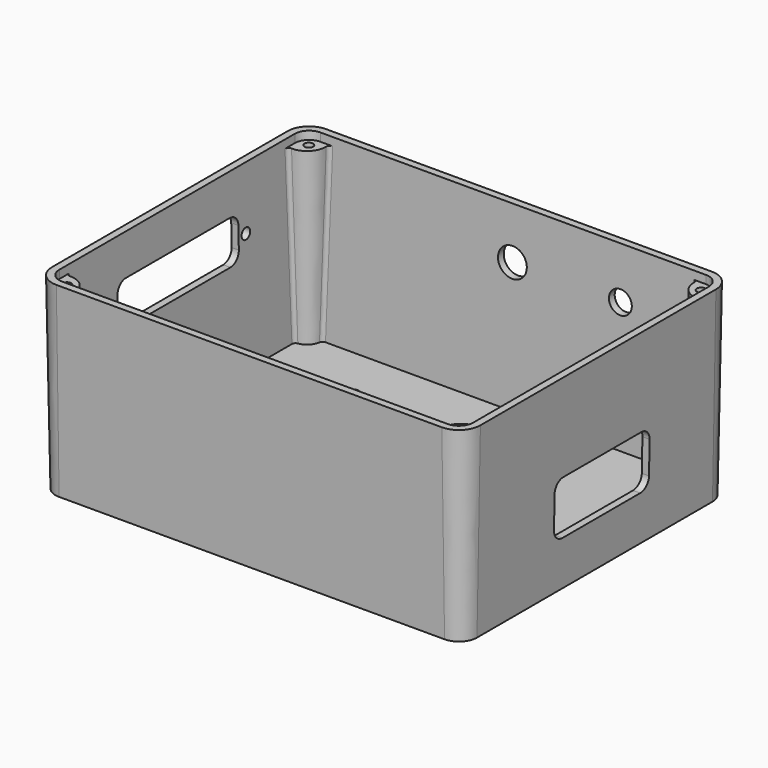
from build123d import *

# Parameters (mm, degrees)
F1_DEPTH                  = 52.25
F1_TAPER                  = -1.05
F2_T                      = 2
F4_D                      = 3
F4_CSINK_D                = 6.5
F4_CSINK_ANGLE            = 90
F6_REACH                  = 95.7577764887
F7_R                      = 1.5
F8_REACH                  = 103.1892979036
F9_R                      = 4
F9_R_2                    = 3.175
F10_REACH                 = 58.1723470669
F12_DEPTH                 = 48
DRAFT_F12_DRAFTED_ANGLE   = -1.5
DRAFT_F12_2_DRAFTED_ANGLE = -1.5
DRAFT_F12_3_DRAFTED_ANGLE = -1.5
DRAFT_F12_4_DRAFTED_ANGLE = -1.5
F13_R                     = 1
F15_D                     = 2.4
F15_DEPTH                 = 8
F15_TIP                   = 0.7210327428


# Not quite as in the source:
# - an extrude with a draft is written as a straight extrude whose walls are then drafted
# - a shell that OpenCascade refuses in one call is made with other operations: the cavity is built on its own and cut out


with BuildPart() as f1:
    # F0 (on Top) → F1 (new body)
    with BuildSketch(Plane.XY):
        with BuildLine():
            ThreePointArc((58.55, 40.9), (57.0855339059, 44.4355339059), (53.55, 45.9))
            Line((53.55, 45.9), (-53.55, 45.9))
            ThreePointArc((-53.55, 45.9), (-57.0855339059, 44.4355339059), (-58.55, 40.9))
            Line((-58.55, 40.9), (-58.55, -40.9))
            ThreePointArc((-58.55, -40.9), (-57.0855339059, -44.4355339059), (-53.55, -45.9))
            Line((-53.55, -45.9), (53.55, -45.9))
            ThreePointArc((53.55, -45.9), (57.0855339059, -44.4355339059), (58.55, -40.9))
            Line((58.55, -40.9), (58.55, 40.9))
        make_face()
    extrude(amount=F1_DEPTH, taper=F1_TAPER)

    # F2: shell of thickness 2, made by hand


with BuildPart() as f2_core1:
    # F2_t2: copy of F1
    add(f1.part)

    # the walls: a layer under each face that stays
    f2_faces = [f2_core1.faces().sort_by_distance(p)[0] for p in [
        (59.028819234, 0, 26.125),
        (57.4241102332, 44.7741102332, 26.125),
        (0, 46.378819234, 26.125),
        (-57.4241102332, 44.7741102332, 26.125),
        (-59.028819234, 0, 26.125),
        (-57.4241102332, -44.7741102332, 26.125),
        (0, -46.378819234, 26.125),
        (57.4241102332, -44.7741102332, 26.125),
        (0, 0, 0),
    ]]
    thicken(f2_faces, amount=-F2_T, mode=Mode.SUBTRACT)


with BuildPart() as f1_1:
    add(f1.part)

    # what is left inside the walls is the cavity
    f2_cavity = [f2_core1.part.solids().sort_by_distance(p)[0] for p in [
        (0, -14.952434, 52.23),
    ]]
    add(f2_cavity, mode=Mode.SUBTRACT)

    # F4 (through all)
    with Locations(Plane(origin=(0, 0, 0), x_dir=(1, 0, 0), z_dir=(0, 0, -1))):
        with Locations((50.05, 21.25), (50.05, -29.25), (-31.865, -29.25), (-31.865, 21.25)):
            CounterSinkHole(F4_D / 2, F4_CSINK_D / 2, counter_sink_angle=F4_CSINK_ANGLE)

    f6_end = f1_1.faces().sort_by_distance((59.028819234, 0, 26.125))[0]
    # F5 (on Right) → F6 (cut, up to a face of the model that its end follows)
    with BuildSketch(Plane.YZ):
        with BuildLine():
            Line((-11.5, 12.5), (15.5, 12.5))
            ThreePointArc((15.5, 12.5), (17.6213203436, 13.3786796564), (18.5, 15.5))
            Line((18.5, 15.5), (18.5, 24.5))
            ThreePointArc((18.5, 24.5), (17.6213203436, 26.6213203436), (15.5, 27.5))
            Line((15.5, 27.5), (-11.5, 27.5))
            ThreePointArc((-11.5, 27.5), (-13.6213203436, 26.6213203436), (-14.5, 24.5))
            Line((-14.5, 24.5), (-14.5, 15.5))
            ThreePointArc((-14.5, 15.5), (-13.6213203436, 13.3786796564), (-11.5, 12.5))
        make_face()
    f6_long = extrude(amount=F6_REACH, mode=Mode.PRIVATE)
    add(split(f6_long, bisect_by=f6_end, keep=Keep.BOTTOM, mode=Mode.PRIVATE), mode=Mode.SUBTRACT)

    f8_end = f1_1.faces().sort_by_distance((-59.028819234, 0, 26.125))[0]
    # F7 (on Right) → F8 (cut, up to a face of the model that its end follows)
    with BuildSketch(Plane.YZ):
        with BuildLine():
            ThreePointArc((21, 38), (20.1213203436, 40.1213203436), (18, 41))
            Line((18, 41), (-18, 41))
            ThreePointArc((-18, 41), (-20.1213203436, 40.1213203436), (-21, 38))
            Line((-21, 38), (-21, 32))
            ThreePointArc((-21, 32), (-20.1213203436, 29.8786796564), (-18, 29))
            Line((-18, 29), (18, 29))
            ThreePointArc((18, 29), (20.1213203436, 29.8786796564), (21, 32))
            Line((21, 32), (21, 38))
        make_face()
        with Locations((-23.52, 35)):
            Circle(F7_R)
        with Locations((23.52, 35)):
            Circle(F7_R)
    f8_long = extrude(amount=-F8_REACH, mode=Mode.PRIVATE)
    add(split(f8_long, bisect_by=f8_end, keep=Keep.BOTTOM, mode=Mode.PRIVATE), mode=Mode.SUBTRACT)

    f10_end = f1_1.faces().sort_by_distance((0, 46.378819234, 26.125))[0]
    # F9 (on Front) → F10 (cut, up to a face of the model that its end follows)
    with BuildSketch(Plane.XZ):
        with Locations((0, 38)):
            Circle(F9_R)
        with Locations((30, 38)):
            Circle(F9_R_2)
    f10_long = extrude(amount=-F10_REACH, mode=Mode.PRIVATE)
    add(split(f10_long, bisect_by=f10_end, keep=Keep.BOTTOM, mode=Mode.PRIVATE), mode=Mode.SUBTRACT)


with BuildPart() as f12_drafted:
    # F11 (on face) → F12 (new body)
    with BuildSketch(Plane.XY.offset(2)):
        with BuildLine():
            Line((-56.5863201302, 40.9), (-56.5863201302, 39.7053273134))
            ThreePointArc((-56.5863201302, 39.7053273134), (-53.5198083649, 40.8698083649), (-52.3553273134, 43.9363201302))
            Line((-52.3553273134, 43.9363201302), (-53.55, 43.9363201302))
            ThreePointArc((-53.55, 43.9363201302), (-55.6970025539, 43.0470025539), (-56.5863201302, 40.9))
        make_face()
    extrude(amount=F12_DEPTH)

    # draft_F12_drafted
    draft_f12_drafted_walls = [f12_drafted.faces().sort_by_distance(p)[0] for p in [
        (-56.5863201302, 40.3026636567, 34),
        (-53.5198083649, 40.8698083649, 34),
        (-52.9526636567, 43.9363201302, 34),
        (-55.6970025539, 43.0470025539, 34),
    ]]
    draft(draft_f12_drafted_walls, neutral_plane=Plane.XY.offset(2), angle=DRAFT_F12_DRAFTED_ANGLE)


with BuildPart() as f1_2:
    add(f1_1.part)

    # join_F12_drafted: union F12_drafted
    add(f12_drafted.part)


with BuildPart() as f12_2_drafted:
    # F11 (on face) → F12, piece 2 (new body)
    with BuildSketch(Plane.XY.offset(2)):
        with BuildLine():
            Line((53.55, 43.9363201302), (52.3553273134, 43.9363201302))
            ThreePointArc((52.3553273134, 43.9363201302), (53.5198083649, 40.8698083649), (56.5863201302, 39.7053273134))
            Line((56.5863201302, 39.7053273134), (56.5863201302, 40.9))
            ThreePointArc((56.5863201302, 40.9), (55.6970025539, 43.0470025539), (53.55, 43.9363201302))
        make_face()
    extrude(amount=F12_DEPTH)

    # draft_F12_2_drafted
    draft_f12_2_drafted_walls = [f12_2_drafted.faces().sort_by_distance(p)[0] for p in [
        (52.9526636567, 43.9363201302, 34),
        (53.5198083649, 40.8698083649, 34),
        (56.5863201302, 40.3026636567, 34),
        (55.6970025539, 43.0470025539, 34),
    ]]
    draft(draft_f12_2_drafted_walls, neutral_plane=Plane.XY.offset(2), angle=DRAFT_F12_2_DRAFTED_ANGLE)


with BuildPart() as f1_3:
    add(f1_2.part)

    # join_F12_2_drafted: union F12_2_drafted
    add(f12_2_drafted.part)


with BuildPart() as f12_3_drafted:
    # F11 (on face) → F12, piece 3 (new body)
    with BuildSketch(Plane.XY.offset(2)):
        with BuildLine():
            ThreePointArc((56.5863201302, -39.7053273134), (53.5198083649, -40.8698083649), (52.3553273134, -43.9363201302))
            Line((52.3553273134, -43.9363201302), (53.55, -43.9363201302))
            ThreePointArc((53.55, -43.9363201302), (55.6970025539, -43.0470025539), (56.5863201302, -40.9))
            Line((56.5863201302, -40.9), (56.5863201302, -39.7053273134))
        make_face()
    extrude(amount=F12_DEPTH)

    # draft_F12_3_drafted
    draft_f12_3_drafted_walls = [f12_3_drafted.faces().sort_by_distance(p)[0] for p in [
        (56.5863201302, -40.3026636567, 34),
        (53.5198083649, -40.8698083649, 34),
        (52.9526636567, -43.9363201302, 34),
        (55.6970025539, -43.0470025539, 34),
    ]]
    draft(draft_f12_3_drafted_walls, neutral_plane=Plane.XY.offset(2), angle=DRAFT_F12_3_DRAFTED_ANGLE)


with BuildPart() as f1_4:
    add(f1_3.part)

    # join_F12_3_drafted: union F12_3_drafted
    add(f12_3_drafted.part)


with BuildPart() as f12_4_drafted:
    # F11 (on face) → F12, piece 4 (new body)
    with BuildSketch(Plane.XY.offset(2)):
        with BuildLine():
            ThreePointArc((-52.3553273134, -43.9363201302), (-53.5198083649, -40.8698083649), (-56.5863201302, -39.7053273134))
            Line((-56.5863201302, -39.7053273134), (-56.5863201302, -40.9))
            ThreePointArc((-56.5863201302, -40.9), (-55.6970025539, -43.0470025539), (-53.55, -43.9363201302))
            Line((-53.55, -43.9363201302), (-52.3553273134, -43.9363201302))
        make_face()
    extrude(amount=F12_DEPTH)

    # draft_F12_4_drafted
    draft_f12_4_drafted_walls = [f12_4_drafted.faces().sort_by_distance(p)[0] for p in [
        (-52.9526636567, -43.9363201302, 34),
        (-53.5198083649, -40.8698083649, 34),
        (-56.5863201302, -40.3026636567, 34),
        (-55.6970025539, -43.0470025539, 34),
    ]]
    draft(draft_f12_4_drafted_walls, neutral_plane=Plane.XY.offset(2), angle=DRAFT_F12_4_DRAFTED_ANGLE)


with BuildPart() as f1_5:
    add(f1_4.part)

    # join_F12_4_drafted: union F12_4_drafted
    add(f12_4_drafted.part)

    # F13
    f13_edges = [f1_5.edges().sort_by_distance(p)[0] for p in [
        (51.769702, 44.376186, 25.999672),
        (57.026186, 39.119702, 25.999672),
        (57.026186, -39.119702, 25.999672),
        (51.769702, -44.376186, 25.999672),
        (-51.769702, -44.376186, 25.999672),
        (-57.026186, -39.119702, 25.999672),
        (-57.026186, 39.119702, 25.999672),
        (-51.769702, 44.376186, 25.999672),
    ]]
    fillet(f13_edges, radius=F13_R)

    # F15
    with Locations(Plane.XY.offset(50)):
        with Locations((-54.5, 42), (54.5, 42), (54.5, -42), (-54.5, -42)):
            Hole(F15_D / 2, depth=F15_DEPTH)
            with Locations((0, 0, -(F15_DEPTH + F15_TIP / 2))):  # 118° drill point
                Cone(0, F15_D / 2, F15_TIP, mode=Mode.SUBTRACT)


solid = f1_5.part
